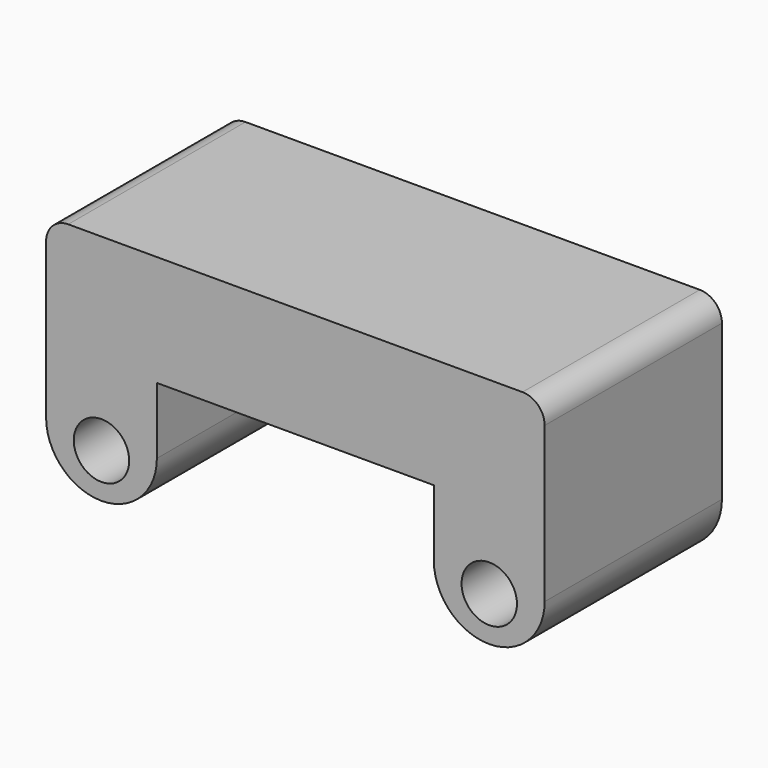
from build123d import *

# Parameters (mm, degrees)
F0_R     = 2.5
F1_DEPTH = 20
F2_R     = 4.99999
F3_R     = 2


# Not quite as in the source:
# - a fillet or chamfer is up to 0.001 mm smaller than in the source, because OpenCascade refuses the exact size


with BuildPart() as f1:
    # F0 (on Front) → F1 (new body)
    with BuildSketch(Plane.XZ):
        Polygon((22.5, 10.5), (-22.5, 10.5), (-22.5, -10.5), (-12.5, -10.5), (-12.5, 0.5), (12.5, 0.5), (12.5, -10.5), (22.5, -10.5), align=None)
        with Locations((-17.5, -6.5)):
            Circle(F0_R, mode=Mode.SUBTRACT)
        with Locations((17.5, -6.5)):
            Circle(F0_R, mode=Mode.SUBTRACT)
    extrude(amount=F1_DEPTH)

    # F2 (radius 5 in the source; OpenCascade refuses exactly that, so slightly less here)
    f2_edges = [f1.edges().sort_by_distance(p)[0] for p in [
        (-22.5, -10, -10.5),
        (-12.5, -10, -10.5),
        (12.5, -10, -10.5),
        (22.5, -10, -10.5),
    ]]
    fillet(f2_edges, radius=F2_R)

    # F3
    f3_edges = [f1.edges().sort_by_distance(p)[0] for p in [
        (22.5, -10, 10.5),
        (-22.5, -10, 10.5),
    ]]
    fillet(f3_edges, radius=F3_R)


solid = f1.part
